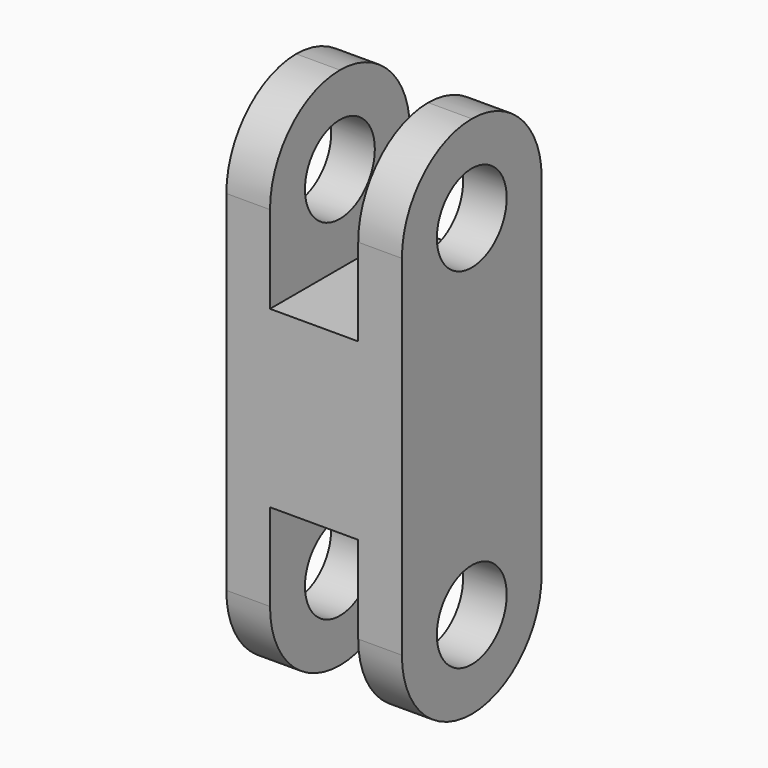
from build123d import *

# Parameters (mm, degrees)
F0_W      = 40
F0_H      = 80
F1_DEPTH  = 20.1
F2_W      = 40
F2_H      = 40
F3_DEPTH  = 10
F4_R      = 10
F5_DEPTH  = 10.1
F7_R      = 19.99999
F8_R      = 10
F9_DEPTH  = 80
F10_W     = 20.2
F10_H     = 40
F11_DEPTH = 40
F12_R     = 19.99999


# Not quite as in the source:
# - a fillet or chamfer is up to 0.001 mm smaller than in the source, because OpenCascade refuses the exact size


with BuildPart() as f1:
    # F0 (on Right) → F1 (new body)
    with BuildSketch(Plane.YZ):
        Rectangle(F0_W, F0_H)
    extrude(amount=F1_DEPTH)

    # F2 (on face) → F3 (join)
    with BuildSketch(Plane.YZ.offset(20.1)):
        with Locations((0, 60)):
            Rectangle(F2_W, F2_H)
    extrude(amount=-F3_DEPTH)

    # F4 (on face) → F5 (cut)
    with BuildSketch(Plane.YZ.offset(20.1)):
        with Locations((0, 60)):
            Circle(F4_R)
    extrude(amount=-F5_DEPTH, mode=Mode.SUBTRACT)

    # F6: F1 across face


with BuildPart() as f1_1:
    add(f1.part)
    add(f1.part.mirror(Plane(origin=(0, 0, 0), x_dir=(0, 1, 0), z_dir=(-1, 0, 0))))

    # F7 (radius 20 in the source; OpenCascade refuses exactly that, so slightly less here)
    f7_edges = [f1_1.edges().sort_by_distance(p)[0] for p in [
        (15.1, 20, 80),
        (15.1, -20, 80),
        (-15.1, 20, 80),
        (-15.1, -20, 80),
    ]]
    fillet(f7_edges, radius=F7_R)

    # F8 (on face) → F9 (cut)
    with BuildSketch(Plane(origin=(-20.1, 0, 0), x_dir=(0, -1, 0), z_dir=(-1, 0, 0))):
        with Locations((0, -20)):
            Circle(F8_R)
    extrude(amount=-F9_DEPTH, mode=Mode.SUBTRACT)

    # F10 (on face) → F11 (cut, through all)
    with BuildSketch(Plane(origin=(0, 20, 0), x_dir=(-1, 0, 0), z_dir=(0, 1, 0))):
        with Locations((0, -20)):
            Rectangle(F10_W, F10_H)
    extrude(amount=-F11_DEPTH, mode=Mode.SUBTRACT)

    # F12 (radius 20 in the source; OpenCascade refuses exactly that, so slightly less here)
    f12_edges = [f1_1.edges().sort_by_distance(p)[0] for p in [
        (-15.1, 20, -40),
        (-15.1, -20, -40),
        (15.1, 20, -40),
        (15.1, -20, -40),
    ]]
    fillet(f12_edges, radius=F12_R)


solid = f1_1.part
